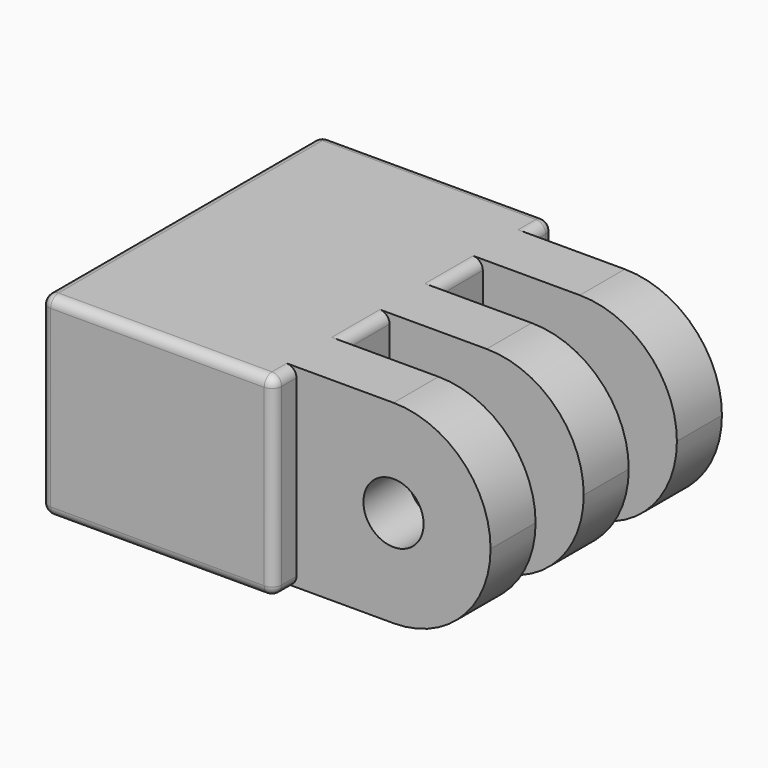
from build123d import *

# Parameters (mm, degrees)
F0_W     = 10
F0_H     = 2.9
F1_DEPTH = 10
F2_R     = 3.05
F3_DEPTH = 8
F4_R     = 1.55
F5_DEPTH = 25
F6_R     = 0.5
F7_R     = 4.99999


# Not quite as in the source:
# - a fillet or chamfer is up to 0.001 mm smaller than in the source, because OpenCascade refuses the exact size


with BuildPart() as f1:
    # F0 (on Top) → F1 (new body)
    with BuildSketch(Plane.XY):
        Polygon((6, 9), (-6, 9), (-6, -9), (6, -9), (6, -7.55), (6, -4.65), (6, -1.55), (6, 1.35), (6, 4.45), (6, 7.35), align=None)
        with Locations((11, 5.9)):
            Rectangle(F0_W, F0_H)
        with Locations((11, -0.1)):
            Rectangle(F0_W, F0_H)
        with Locations((11, -6.1)):
            Rectangle(F0_W, F0_H)
    extrude(amount=F1_DEPTH)

    # F2 (on face) → F3 (cut)
    with BuildSketch(Plane(origin=(-6, 0, 0), x_dir=(0, -1, 0), z_dir=(-1, 0, 0))):
        with Locations((0, 5)):
            Circle(F2_R)
    extrude(amount=-F3_DEPTH, mode=Mode.SUBTRACT)

    # F4 (on face) → F5 (cut)
    with BuildSketch(Plane.XZ.offset(7.55)):
        with Locations((11, 5)):
            Circle(F4_R)
    extrude(amount=-F5_DEPTH, mode=Mode.SUBTRACT)

    # F6
    f6_edges = [f1.edges().sort_by_distance(p)[0] for p in [
        (-6, 0, 10),
        (0, -9, 10),
        (0, 9, 10),
        (-6, -9, 5),
        (-6, 0, 0),
        (-6, 9, 5),
        (0, 9, 0),
        (0, -9, 0),
        (6, -9, 5),
        (6, -8.275, 0),
        (6, -3.1, 0),
        (6, 2.9, 0),
        (6, 8.175, 0),
        (6, 9, 5),
        (6, 8.175, 10),
        (6, 2.9, 10),
        (6, -3.1, 10),
        (6, -8.275, 10),
    ]]
    fillet(f6_edges, radius=F6_R)

    # F7 (radius 5 in the source; OpenCascade refuses exactly that, so slightly less here)
    f7_edges = [f1.edges().sort_by_distance(p)[0] for p in [
        (16, 5.9, 0),
        (16, 5.9, 10),
        (16, -0.1, 10),
        (16, -0.1, 0),
        (16, -6.1, 0),
        (16, -6.1, 10),
    ]]
    fillet(f7_edges, radius=F7_R)


solid = f1.part
